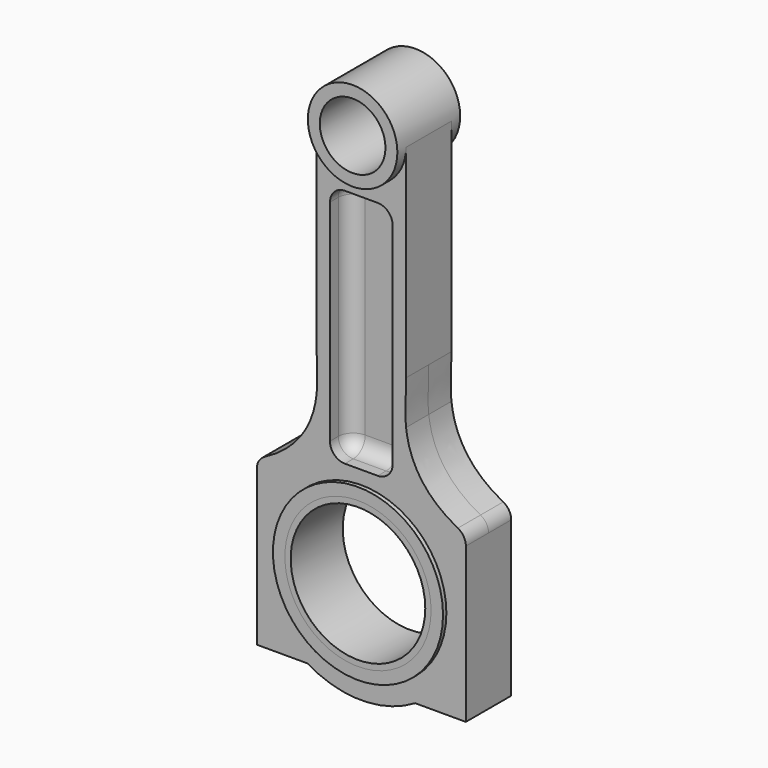
from build123d import *

# Parameters (mm, degrees)
F0_R     = 28.5
F1_DEPTH = 9.5
F0_R_2   = 24.5
F2_DEPTH = 10.9
F0_R_3   = 11
F3_DEPTH = 13.15
F0_R_4   = 22.55
F4_DEPTH = 10.9
F6_DEPTH = 8.5
F7_R     = 5
F9_R     = 5


# Not quite as in the source:
# - a feature of the source that left no trace in its solid (it failed there, or was rolled back) is left out
# - a pattern or mirror of a feature is missing from the dataset's text; its kind, count and spacing are read off the source's solid


with BuildPart() as f1:
    # F0 (on Front) → F1 (new body, symmetric)
    with BuildSketch(Plane.XZ):
        with BuildLine():
            Line((15, 65), (15, 133))
            ThreePointArc((15, 133), (0, 118), (-15, 133))
            Line((-15, 133), (-15, 65))
            add(Edge.make_bspline(
                [(-15, 65), (-15, 56.7374224028), (-14.4979846104, 54.6858215893), (-15, 50.3263995051)],
                knots=[0, 0, 0, 0, 0.4026758, 0.4026758, 0.4026758, 0.4026758], degree=3))
            Line((-15, 50.3263995051), (-15, 31.6227766017))
            ThreePointArc((-15, 31.6227766017), (0, 35), (15, 31.6227766017))
            Line((15, 31.6227766017), (15, 50.3263995051))
            add(Edge.make_bspline(
                [(15, 65), (15, 56.7374224028), (14.4979846104, 54.6858215893), (15, 50.3263995051)],
                knots=[0, 0, 0, 0, 0.4026758, 0.4026758, 0.4026758, 0.4026758], degree=3))
        make_face()
        with BuildLine():
            Line((-15, 31.6227766017), (-15, 50.3263995051))
            add(Edge.make_bspline(
                [(-15, 50.3263995051), (-15.7446832935, 43.8596878017), (-18.6986741861, 32.3147582025), (-35.0277563773, 25)],
                knots=[0.4026758, 0.4026758, 0.4026758, 0.4026758, 1, 1, 1, 1], degree=3))
            Line((-35.0277563773, 25), (-35.0277563773, -30))
            Line((-35.0277563773, -30), (-18.0277563773, -30))
            ThreePointArc((-18.0277563773, -30), (-34.9578291925, 1.7176082629), (-15, 31.6227766017))
        make_face()
        with BuildLine():
            add(Edge.make_bspline(
                [(15, 50.3263995051), (15.7446832935, 43.8596878017), (18.6986741861, 32.3147582025), (35.0277563773, 25)],
                knots=[0.4026758, 0.4026758, 0.4026758, 0.4026758, 1, 1, 1, 1], degree=3))
            Line((15, 50.3263995051), (15, 31.6227766017))
            ThreePointArc((15, 31.6227766017), (29.5803989155, 18.7082869339), (35, 0))
            ThreePointArc((35, 0), (30.4628583131, -17.2341017578), (18.0277563773, -30))
            Line((18.0277563773, -30), (35.0277563773, -30))
            Line((35.0277563773, -30), (35.0277563773, 25))
        make_face()
        with BuildLine():
            ThreePointArc((35, 0), (29.5803989155, 18.7082869339), (15, 31.6227766017))
            ThreePointArc((15, 31.6227766017), (0, 35), (-15, 31.6227766017))
            ThreePointArc((-15, 31.6227766017), (-34.9578291925, 1.7176082629), (-18.0277563773, -30))
            ThreePointArc((-18.0277563773, -30), (0, -35), (18.0277563773, -30))
            ThreePointArc((18.0277563773, -30), (30.4628583131, -17.2341017578), (35, 0))
        make_face()
        Circle(F0_R, mode=Mode.SUBTRACT)
    extrude(amount=F1_DEPTH, both=True)

    # F0 (on Front) → F2 (join, symmetric)
    with BuildSketch(Plane.XZ):
        Circle(F0_R)
        Circle(F0_R_2, mode=Mode.SUBTRACT)
    extrude(amount=F2_DEPTH, both=True)

    # F0 (on Front) → F3 (join, symmetric)
    with BuildSketch(Plane.XZ):
        with BuildLine():
            ThreePointArc((-15, 133), (0, 118), (15, 133))
            ThreePointArc((15, 133), (0, 148), (-15, 133))
        make_face()
        with Locations((0, 133)):
            Circle(F0_R_3, mode=Mode.SUBTRACT)
    extrude(amount=F3_DEPTH, both=True)

    # F5 (on face) → F6 (cut)
    with BuildSketch(Plane.XZ.offset(9.5)):
        with BuildLine():
            Line((5.5, 113.5), (-5.5, 113.5))
            ThreePointArc((-5.5, 113.5), (-9.0355339059, 112.0355339059), (-10.5, 108.5))
            Line((-10.5, 108.5), (-10.5, 38))
            ThreePointArc((-10.5, 38), (-9.0355339059, 34.4644660941), (-5.5, 33))
            Line((-5.5, 33), (5.5, 33))
            ThreePointArc((5.5, 33), (9.0355339059, 34.4644660941), (10.5, 38))
            Line((10.5, 38), (10.5, 108.5))
            ThreePointArc((10.5, 108.5), (9.0355339059, 112.0355339059), (5.5, 113.5))
        make_face()
    f6 = extrude(amount=-F6_DEPTH, mode=Mode.SUBTRACT)

    # F6_copies: F6 across plane
    add(f6.mirror(Plane.ZX), mode=Mode.SUBTRACT)

    # F7
    f7_edges = [f1.edges().sort_by_distance(p)[0] for p in [
        (10.5, -1, 73.25),
        (0, -1, 113.5),
        (9.035534, -1, 112.035534),
        (-9.035534, -1, 112.035534),
        (-10.5, -1, 73.25),
        (-9.035534, -1, 34.464466),
        (0, -1, 33),
        (9.035534, -1, 34.464466),
    ]]
    fillet(f7_edges, radius=F7_R)

    # F9
    f9_edges = [f1.edges().sort_by_distance(p)[0] for p in [
        (35.027756, -4.75, 25),
        (35.027756, 4.75, 25),
        (-35.027756, -4.75, 25),
        (-35.027756, 4.75, 25),
        (9.035534, 1, 112.035534),
        (0, 1, 113.5),
        (-9.035534, 1, 112.035534),
        (-10.5, 1, 73.25),
        (-9.035534, 1, 34.464466),
        (0, 1, 33),
        (9.035534, 1, 34.464466),
        (10.5, 1, 73.25),
    ]]
    fillet(f9_edges, radius=F9_R)


with BuildPart() as f4:
    # F0 (on Front) → F4 (new body, symmetric)
    with BuildSketch(Plane.XZ):
        Circle(F0_R_2)
        Circle(F0_R_4, mode=Mode.SUBTRACT)
    extrude(amount=F4_DEPTH, both=True)


solid = Compound([f1.part, f4.part])
